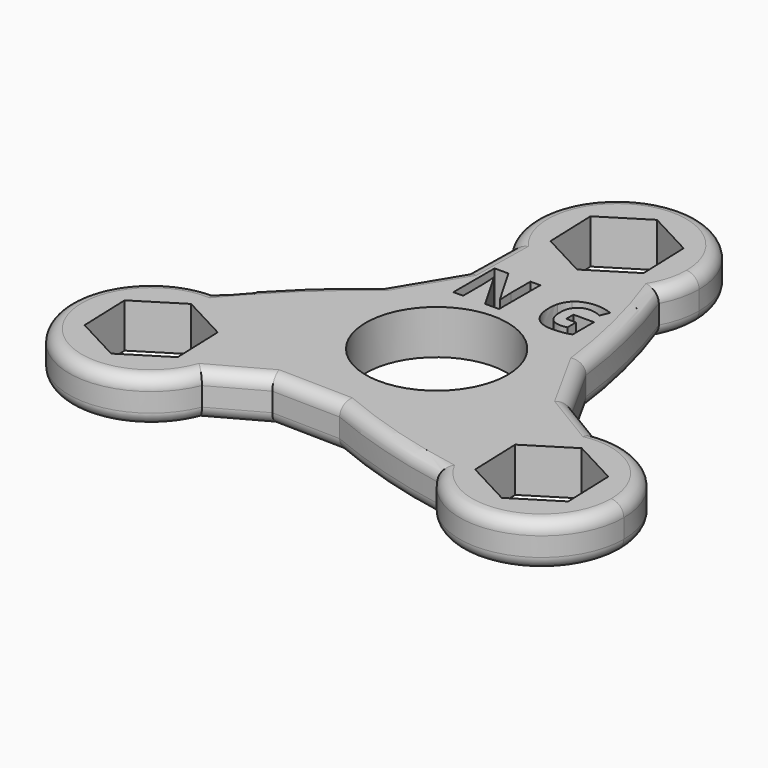
from build123d import *

# Parameters (mm, degrees)
F0_R     = 11.2
F1_DEPTH = 7
F2_R     = 2
F3_R     = 2


with BuildPart() as f1:
    # F0 (on Top) → F1 (new body)
    with BuildSketch(Plane.XY):
        with BuildLine():
            ThreePointArc((12.974149, 35.662882), (-4.177163, 47.946198), (-10.284386, 27.753398))
            ThreePointArc((-10.284386, 27.753398), (1.089699, 22.734576), (11.463228, 29.586457))
            ThreePointArc((11.463228, 29.586457), (12.590754, 32.532155), (12.974149, 35.662882))
        make_face()
        Polygon((-7.016451, 31.277602), (-7.305989, 39.546667), (-0.289539, 43.931947), (7.016451, 40.048162), (7.305989, 31.779097), (0.289539, 27.393817), align=None, mode=Mode.SUBTRACT)
        with BuildLine():
            Line((-2.182666, 18.780464), (-4.253872, 18.820335))
            Line((-4.253872, 18.820335), (-2.138071, 15.171006))
            Line((-2.138071, 15.171006), (-2.098828, 15.171006))
            add(Edge.make_bspline(
                [(-2.098828, 15.171006), (-2.182666, 16.760362), (-2.182666, 17.416796)],
                knots=[0, 0, 0, 1, 1, 1], degree=2))
            Line((-2.182666, 17.416796), (-2.182666, 18.780464))
        make_face()
        with BuildLine():
            Line((-16.041666, 9.67803), (-21.62928, 0.41637))
            Line((-21.62928, 0.41637), (-11.175227, -18.523321))
            Line((-11.175227, -18.523321), (-0.360587, -18.731506))
            Line((-0.360587, -18.731506), (10.454053, -18.939691))
            Line((10.454053, -18.939691), (21.62928, -0.41637))
            Line((21.62928, -0.41637), (16.402253, 9.053475))
            Line((16.402253, 9.053475), (11.175227, 18.523321))
            Line((11.175227, 18.523321), (6.096901, 18.62108))
            add(Edge.make_bspline(
                [(6.096901, 18.62108), (5.806924, 18.010659), (5.806924, 17.177769)],
                knots=[0.34421, 0.34421, 0.34421, 1, 1, 1], degree=2))
            add(Edge.make_bspline(
                [(5.806924, 17.177769), (5.806924, 15.85063), (6.350087, 15.151385)],
                knots=[0, 0, 0, 1, 1, 1], degree=2))
            add(Edge.make_bspline(
                [(6.350087, 15.151385), (6.893251, 14.452139), (7.929632, 14.452139)],
                knots=[0, 0, 0, 1, 1, 1], degree=2))
            add(Edge.make_bspline(
                [(7.929632, 14.452139), (8.471904, 14.452139), (9.028446, 14.562734)],
                knots=[0, 0, 0, 1, 1, 1], degree=2))
            Line((9.028446, 14.562734), (9.028446, 16.262685))
            Line((9.028446, 16.262685), (7.483685, 16.262685))
            Line((7.483685, 16.262685), (7.483685, 17.702202))
            Line((7.483685, 17.702202), (10.717694, 17.702202))
            Line((10.717694, 17.702202), (10.717694, 13.476407))
            add(Edge.make_bspline(
                [(10.717694, 13.476407), (9.931043, 13.219541), (9.237149, 13.116082)],
                knots=[0, 0, 0, 1, 1, 1], degree=2))
            add(Edge.make_bspline(
                [(9.237149, 13.116082), (8.543255, 13.012622), (7.819037, 13.012622)],
                knots=[0, 0, 0, 1, 1, 1], degree=2))
            add(Edge.make_bspline(
                [(7.819037, 13.012622), (5.9746, 13.012622), (5.001543, 14.097165)],
                knots=[0, 0, 0, 1, 1, 1], degree=2))
            add(Edge.make_bspline(
                [(5.001543, 14.097165), (4.028486, 15.181709), (4.028486, 17.21166)],
                knots=[0, 0, 0, 1, 1, 1], degree=2))
            add(Edge.make_bspline(
                [(4.028486, 17.21166), (4.028486, 18.004795), (4.210978, 18.657385)],
                knots=[0, 0, 0, 0.402021, 0.402021, 0.402021], degree=2))
            Line((4.210978, 18.657385), (-0.627202, 18.750521))
            Line((-0.627202, 18.750521), (-0.627202, 13.125001))
            Line((-0.627202, 13.125001), (-2.823046, 13.125001))
            Line((-2.823046, 13.125001), (-6.119845, 18.856256))
            Line((-6.119845, 18.856256), (-6.391933, 18.861494))
            add(Edge.make_bspline(
                [(-6.391933, 18.861494), (-6.312137, 17.562378), (-6.312137, 16.960146)],
                knots=[0.136538, 0.136538, 0.136538, 1, 1, 1], degree=2))
            Line((-6.312137, 16.960146), (-6.312137, 13.125001))
            Line((-6.312137, 13.125001), (-7.856898, 13.125001))
            Line((-7.856898, 13.125001), (-7.856898, 18.889695))
            Line((-7.856898, 18.889695), (-10.454053, 18.939691))
            Line((-10.454053, 18.939691), (-16.041666, 9.67803))
        make_face()
        Circle(F0_R, mode=Mode.SUBTRACT)
        with BuildLine():
            Line((-10.284386, 27.753398), (-10.454053, 18.939691))
            Line((-10.454053, 18.939691), (-7.856898, 18.889695))
            Line((-7.856898, 18.889695), (-7.856898, 21.275131))
            Line((-7.856898, 21.275131), (-5.677108, 21.275131))
            Line((-5.677108, 21.275131), (-4.253872, 18.820335))
            Line((-4.253872, 18.820335), (-2.182666, 18.780464))
            Line((-2.182666, 18.780464), (-2.182666, 21.275131))
            Line((-2.182666, 21.275131), (-0.627202, 21.275131))
            Line((-0.627202, 21.275131), (-0.627202, 18.750521))
            Line((-0.627202, 18.750521), (4.210978, 18.657385))
            add(Edge.make_bspline(
                [(4.210978, 18.657385), (4.482423, 19.628069), (5.157624, 20.287804)],
                knots=[0.402021, 0.402021, 0.402021, 1, 1, 1], degree=2))
            add(Edge.make_bspline(
                [(5.157624, 20.287804), (6.286763, 21.391077), (8.28639, 21.391077)],
                knots=[0, 0, 0, 1, 1, 1], degree=2))
            add(Edge.make_bspline(
                [(8.28639, 21.391077), (9.542177, 21.391077), (10.706991, 20.889833)],
                knots=[0, 0, 0, 1, 1, 1], degree=2))
            Line((10.706991, 20.889833), (10.132611, 19.507397))
            add(Edge.make_bspline(
                [(10.132611, 19.507397), (9.240717, 19.953344), (8.275687, 19.953344)],
                knots=[0, 0, 0, 1, 1, 1], degree=2))
            add(Edge.make_bspline(
                [(8.275687, 19.953344), (7.155468, 19.953344), (6.481196, 19.200585)],
                knots=[0, 0, 0, 1, 1, 1], degree=2))
            add(Edge.make_bspline(
                [(6.481196, 19.200585), (6.249104, 18.941477), (6.096901, 18.62108)],
                knots=[0, 0, 0, 0.34421, 0.34421, 0.34421], degree=2))
            Line((6.096901, 18.62108), (11.175227, 18.523321))
            Line((11.175227, 18.523321), (16.402253, 9.053475))
            ThreePointArc((16.402253, 9.053475), (14.503185, 19.457182), (11.463228, 29.586457))
            ThreePointArc((11.463228, 29.586457), (1.089699, 22.734576), (-10.284386, 27.753398))
        make_face()
        with BuildLine():
            Line((-11.175227, -18.523321), (-21.62928, 0.41637))
            Line((-21.62928, 0.41637), (-16.041666, 9.67803))
            ThreePointArc((-16.041666, 9.67803), (-24.102006, 2.831536), (-31.354238, -4.865782))
            ThreePointArc((-31.354238, -4.865782), (-21.878295, -8.492892), (-17.910813, -17.831441))
            ThreePointArc((-17.910813, -17.831441), (-18.158717, -20.35557), (-18.892955, -22.783239))
            Line((-18.892955, -22.783239), (-11.175227, -18.523321))
        make_face()
        with BuildLine():
            Line((10.454053, -18.939691), (-0.360587, -18.731506))
            ThreePointArc((-0.360587, -18.731506), (9.598821, -22.288718), (19.89101, -24.720675))
            ThreePointArc((19.89101, -24.720675), (19.143871, -12.310995), (29.177341, -4.970159))
            Line((29.177341, -4.970159), (21.62928, -0.41637))
            Line((21.62928, -0.41637), (10.454053, -18.939691))
        make_face()
        with BuildLine():
            ThreePointArc((-17.910813, -17.831441), (-21.878295, -8.492892), (-31.354238, -4.865782))
            ThreePointArc((-31.354238, -4.865782), (-41.536354, -25.239301), (-18.892955, -22.783239))
            ThreePointArc((-18.892955, -22.783239), (-18.158717, -20.35557), (-17.910813, -17.831441))
        make_face()
        Polygon((-30.595423, -26.100506), (-37.901413, -22.216721), (-38.190951, -13.947656), (-31.1745, -9.562376), (-23.868511, -13.446161), (-23.578972, -21.715226), align=None, mode=Mode.SUBTRACT)
        with BuildLine():
            add(Edge.make_bspline(
                [(-6.419164, 19.289774), (-6.404551, 19.066921), (-6.391933, 18.861494)],
                knots=[0, 0, 0, 0.136538, 0.136538, 0.136538], degree=2))
            Line((-6.391933, 18.861494), (-6.119845, 18.856256))
            Line((-6.119845, 18.856256), (-6.369218, 19.289774))
            Line((-6.369218, 19.289774), (-6.419164, 19.289774))
        make_face()
        with BuildLine():
            ThreePointArc((29.177341, -4.970159), (19.143871, -12.310995), (19.89101, -24.720675))
            ThreePointArc((19.89101, -24.720675), (34.469049, -30.300717), (43.85911, -17.831441))
            ThreePointArc((43.85911, -17.831441), (39.434044, -8.072254), (29.177341, -4.970159))
        make_face()
        Polygon((37.901413, -13.446161), (38.190951, -21.715226), (31.1745, -26.100506), (23.868511, -22.216721), (23.578972, -13.947656), (30.595423, -9.562376), align=None, mode=Mode.SUBTRACT)
    extrude(amount=F1_DEPTH)

    # F2
    f2_edges = [f1.edges().sort_by_distance(p)[0] for p in [
        (-1.089699, 48.591188, 7),
        (14.503185, 19.457182, 7),
        (19.015767, 4.318553, 7),
        (25.40331, -2.693265, 7),
        (42.626052, -23.351887, 7),
        (9.598821, -22.288718, 7),
        (-5.767907, -18.627413, 7),
        (-15.034091, -20.65328, 7),
        (-41.536354, -25.239301, 7),
        (-24.102006, 2.831536, 7),
        (-13.24786, 14.308861, 7),
        (-10.36922, 23.346545, 7),
    ]]
    fillet(f2_edges, radius=F2_R)

    # F3
    f3_edges = [f1.edges().sort_by_distance(p)[0] for p in [
        (-41.536354, -25.239301, 0),
        (-15.034091, -20.65328, 0),
        (-5.767907, -18.627413, 0),
        (9.598821, -22.288718, 0),
        (42.626052, -23.351887, 0),
        (25.40331, -2.693265, 0),
        (19.015767, 4.318553, 0),
        (14.503185, 19.457182, 0),
        (-1.089699, 48.591188, 0),
        (-10.36922, 23.346545, 0),
        (-13.24786, 14.308861, 0),
        (-24.102006, 2.831536, 0),
    ]]
    fillet(f3_edges, radius=F3_R)


solid = f1.part
